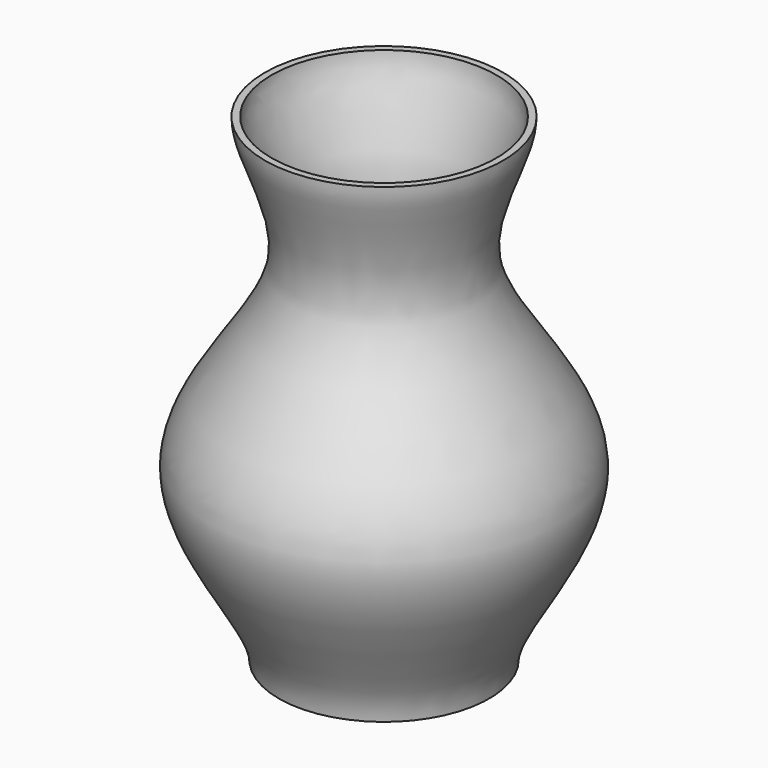
from build123d import *

# Parameters (mm, degrees)
F0_R     = 35.25
F3_DEPTH = 4


# Not quite as in the source:
# - the dataset's text gives a spline's control points without its knots; the knots are read off the source's solid


with BuildPart() as f2:
    # F1 (on Front) → F2 (revolve)
    with BuildSketch(Plane.XZ):
        with BuildLine():
            add(Edge.make_bspline(
                [(-37.4, 0), (-37.4, 14.3522878615), (-87.9725287664, 63.5480280182), (-13.8496681212, 120.2382004241), (-42.3731994979, 159.3802885315), (-42.3731994979, 170.001968361)],
                knots=[0, 0, 0, 0, 0.346394809, 0.7082150898, 1, 1, 1, 1], degree=3))
            Line((-37.4, 0), (-35, 0))
            add(Edge.make_bspline(
                [(-35, 0), (-35, 1.5435615345), (-35.4740709756, 4.6756778265), (-37.1890110114, 9.5372073563), (-39.6421549787, 14.623124194), (-43.6022381632, 21.7081526024), (-48.1697564388, 29.205303647), (-52.4882364896, 36.9284610403), (-55.3877063596, 42.7713468132), (-57.7363520925, 48.5974204314), (-59.0657393891, 53.3749997943), (-59.6613776132, 57.1136107845), (-59.8223125946, 59.4093339667), (-59.8139327523, 61.2198276538), (-59.7152357681, 63.0297922371), (-59.4292640546, 65.2890090559), (-58.8436606367, 68.0021049421), (-57.7640826947, 71.6252558323), (-55.9018093753, 76.1671352682), (-53.0149538831, 81.6318615101), (-48.5416585108, 88.9286602891), (-43.5137019467, 96.2364115739), (-38.7078820067, 103.5947555365), (-35.4107630111, 109.161569174), (-33.0857159356, 113.8650166067), (-31.5853282653, 117.6846071433), (-30.6686341443, 120.5825471763), (-30.1035019872, 123.0266081935), (-29.7869108035, 125.0029181307), (-29.5653294094, 126.9769023682), (-29.4551501007, 129.4343040764), (-29.5940760544, 133.3315419977), (-30.2803192124, 138.1169963171), (-31.6843645256, 143.6733322177), (-33.4430018443, 149.0020378424), (-35.3387323109, 154.056926589), (-37.15804108, 158.7825833299), (-38.6895035826, 163.1084894977), (-39.7281102079, 166.9399913556), (-39.9731994979, 169.0698227633), (-39.9731994979, 170.001968361)],
                knots=[0, 0, 0, 0, 0.03125, 0.0625, 0.09375, 0.125, 0.1875, 0.21875, 0.25, 0.28125, 0.3125, 0.328125, 0.34375, 0.3515625, 0.359375, 0.375, 0.390625, 0.40625, 0.4375, 0.46875, 0.5, 0.5625, 0.59375, 0.625, 0.65625, 0.671875, 0.6875, 0.703125, 0.7109375, 0.71875, 0.734375, 0.75, 0.78125, 0.8125, 0.84375, 0.875, 0.90625, 0.9375, 0.96875, 1, 1, 1, 1], degree=3))
            Line((-39.9731994979, 170.001968361), (-42.3731994979, 170.001968361))
        make_face()
    revolve(axis=Axis((0, 0, 0), (0, 0, 1)))

    # F0 (on Top) → F3 (join)
    with BuildSketch(Plane.XY):
        Circle(F0_R)
    extrude(amount=F3_DEPTH)


solid = f2.part
